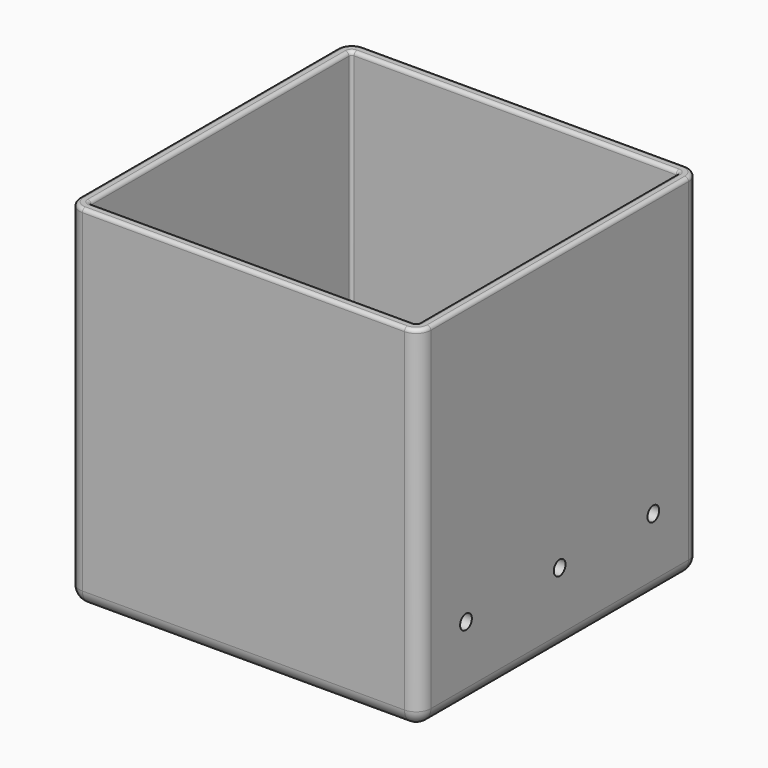
from build123d import *

# Parameters (mm, degrees)
F1_DEPTH     = 76.2
F2_R         = 3.175
F3_T         = -2.54
F4_R         = 1.5875
F5_DEPTH     = 76.201
F6_TEXT_SIZE = 4.4097222222
F7_DEPTH     = 1
F8_R         = 4.7625
F9_DEPTH     = 0.79375
F9_TAPER     = 10
F10_R        = 0.396875
F11_R        = 0.79375


# Not quite as in the source:
# - Text() gives the source's letters only with a copy of the font that has no kerning and outlines rounded to 1/6400 em; it was checked with that copy


with BuildPart() as f1:
    # F0 (on Top) → F1 (new body)
    with BuildSketch(Plane.XY):
        with BuildLine():
            ThreePointArc((76.2, 73.025), (75.2700640303, 75.2700640303), (73.025, 76.2))
            Line((73.025, 76.2), (3.175, 76.2))
            ThreePointArc((3.175, 76.2), (0.9299359697, 75.2700640303), (0, 73.025))
            Line((0, 73.025), (0, 3.175))
            ThreePointArc((0, 3.175), (0.9299359697, 0.9299359697), (3.175, 0))
            Line((3.175, 0), (73.025, 0))
            ThreePointArc((73.025, 0), (75.2700640303, 0.9299359697), (76.2, 3.175))
            Line((76.2, 3.175), (76.2, 73.025))
        make_face()
    extrude(amount=F1_DEPTH)

    # F2
    f2_edges = [f1.edges().sort_by_distance(p)[0] for p in [
        (75.270064, 0.929936, 0),
        (76.2, 38.1, 0),
        (75.270064, 75.270064, 0),
        (38.1, 76.2, 0),
        (0.929936, 75.270064, 0),
        (0, 38.1, 0),
        (0.929936, 0.929936, 0),
        (38.1, 0, 0),
    ]]
    fillet(f2_edges, radius=F2_R)

    # F3
    f3_openings = [f1.faces().sort_by_distance(p)[0] for p in [
        (38.1, 38.1, 76.2),
    ]]
    offset(amount=F3_T, openings=f3_openings)

    # F4 (on face) → F5 (cut, through all)
    with BuildSketch(Plane.YZ.offset(76.2)):
        with Locations((12.7, 15.875)):
            Circle(F4_R)
        with Locations((38.1, 15.875)):
            Circle(F4_R)
        with Locations((63.5, 15.875)):
            Circle(F4_R)
    extrude(amount=-F5_DEPTH, mode=Mode.SUBTRACT)

    # F6 (on face) → F7 (cut)
    with BuildSketch(Plane.XY.offset(2.54)):
        with Locations((9.4598876953, 34.925)):
            Text('3 in SIPP Planter', F6_TEXT_SIZE, font='Open Sans', text_align=(TextAlign.LEFT, TextAlign.BOTTOM))
        with Locations((9.4598876953, 28.9277777778)):
            Text('carnivorous / swamp biome', F6_TEXT_SIZE, font='Open Sans', text_align=(TextAlign.LEFT, TextAlign.BOTTOM))
        with Locations((9.4598876953, 22.9305555556)):
            Text('v0.1', F6_TEXT_SIZE, font='Open Sans', text_align=(TextAlign.LEFT, TextAlign.BOTTOM))
    extrude(amount=-F7_DEPTH, mode=Mode.SUBTRACT)

    # F8 (on face) → F9 (cut)
    with BuildSketch(Plane(origin=(0, 0, 0), x_dir=(1, 0, 0), z_dir=(0, 0, -1))):
        with Locations((11.1125, -11.1125)):
            Circle(F8_R)
        with Locations((65.0875, -11.1125)):
            Circle(F8_R)
        with Locations((11.1125, -65.0875)):
            Circle(F8_R)
        with Locations((65.0875, -65.0875)):
            Circle(F8_R)
    extrude(amount=-F9_DEPTH, taper=F9_TAPER, mode=Mode.SUBTRACT)

    # F10
    f10_edges = [f1.edges().sort_by_distance(p)[0] for p in [
        (6.35, 11.1125, 0),
        (6.35, 65.0875, 0),
        (60.325, 11.1125, 0),
        (60.325, 65.0875, 0),
        (60.46496, 65.0875, 0.79375),
        (60.46496, 11.1125, 0.79375),
        (6.48996, 11.1125, 0.79375),
        (6.48996, 65.0875, 0.79375),
    ]]
    fillet(f10_edges, radius=F10_R)

    # F11
    f11_edges = [f1.edges().sort_by_distance(p)[0] for p in [
        (75.270064, 0.929936, 76.2),
        (76.2, 38.1, 76.2),
        (75.270064, 75.270064, 76.2),
        (38.1, 76.2, 76.2),
        (0.929936, 75.270064, 76.2),
        (0, 38.1, 76.2),
        (0.929936, 0.929936, 76.2),
        (38.1, 0, 76.2),
        (73.474013, 2.725987, 76.2),
        (38.1, 2.54, 76.2),
        (2.725987, 2.725987, 76.2),
        (2.54, 38.1, 76.2),
        (2.725987, 73.474013, 76.2),
        (38.1, 73.66, 76.2),
        (73.474013, 73.474013, 76.2),
        (73.66, 38.1, 76.2),
    ]]
    fillet(f11_edges, radius=F11_R)


solid = f1.part
